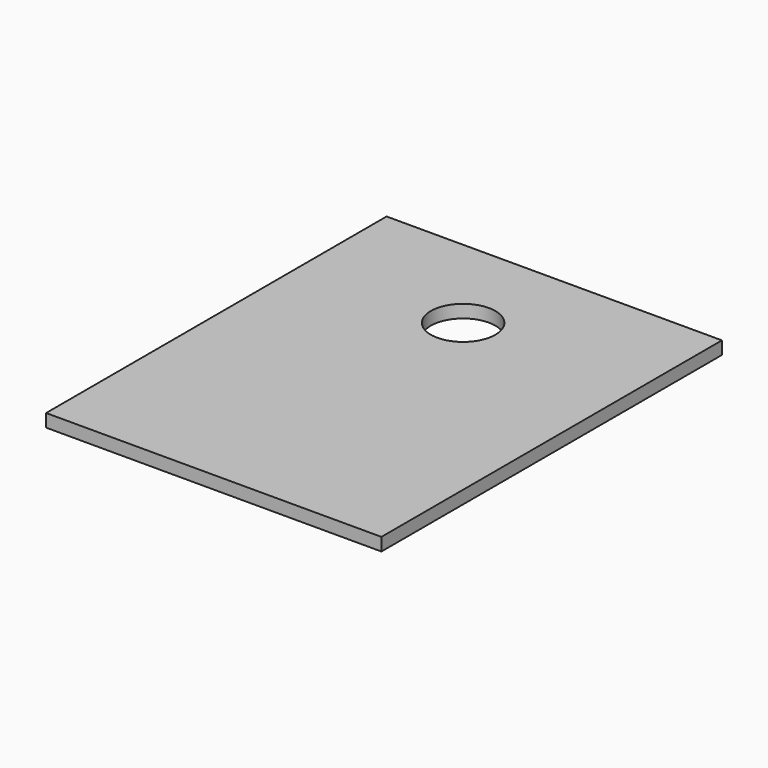
from build123d import *

# Parameters (mm, degrees)
F0_W     = 82.55
F0_H     = 104.775
F1_DEPTH = 3.175
F2_R     = 7.9375
F3_DEPTH = 25.4


# Not quite as in the source:
# - a feature names something its author has since deleted; it is built from what else it names


with BuildPart() as f1:
    # F0 (on Top) → F1 (new body)
    with BuildSketch(Plane.XY):
        with Locations((2.113471739, -26.9875)):
            Rectangle(F0_W, F0_H)
    extrude(amount=F1_DEPTH)

    # F2 (on face) → F3 (cut)
    with BuildSketch(Plane.XY.offset(3.175)):
        Circle(F2_R)
    extrude(amount=-F3_DEPTH, mode=Mode.SUBTRACT)


solid = f1.part
